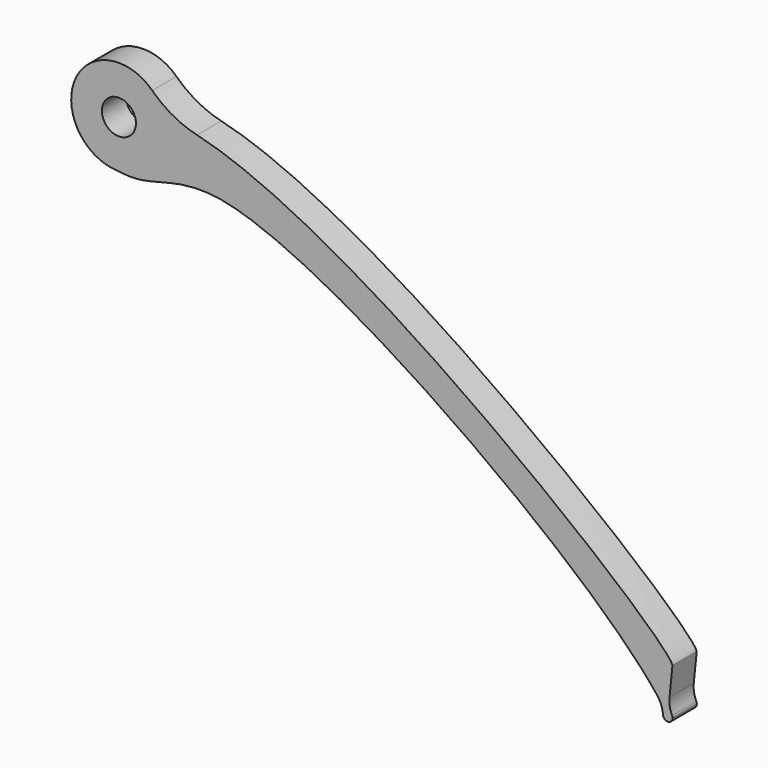
from build123d import *

# Parameters (mm, degrees)
F1_DEPTH = 3.175
F2_R     = 10
F3_R     = 5
F4_R     = 3


# Not quite as in the source:
# - a length typed as a fraction of an inch, garbled in the dataset ("3 / 203.2 mm" for 3/8 in), is restored


with BuildPart() as f1:
    # F0 (on Front) → F1 (new body)
    with BuildSketch(Plane.XZ):
        with BuildLine():
            ThreePointArc((5, 0), (4.9416586843, 0.7615835135), (4.7679962208, 1.5053943132))
            ThreePointArc((4.7679962208, 1.5053943132), (-4.0328012328, 2.9557594992), (0, -5))
            ThreePointArc((0, -5), (3.5355339059, -3.5355339059), (5, 0))
        make_face()
        with BuildLine():
            ThreePointArc((1.4790914289, 1.0009302168), (1.7075036754, 0.5234538686), (1.7859375, 0))
            ThreePointArc((1.7859375, 0), (-1.7075036754, -0.5234538686), (1.4790914289, 1.0009302168))
        make_face(mode=Mode.SUBTRACT)
        with BuildLine():
            add(Edge.make_bspline(
                [(4.7679962208, 1.5053943132), (10.5227651302, 1.3088265612), (33.1362274433, -9.6066408427), (57.5003811193, -30.0100648608), (57.9834021628, -31.7015722394)],
                knots=[0.1250018118, 0.1250018118, 0.1250018118, 0.1250018118, 0.4750790038, 1, 1, 1, 1], degree=3))
            ThreePointArc((4.7679962208, 1.5053943132), (4.9416586843, 0.7615835135), (5, 0))
            ThreePointArc((5, 0), (3.5355339059, -3.5355339059), (0, -5))
            add(Edge.make_bspline(
                [(0, -5), (3.595217635, -5.6845152728), (10.4140448254, 2.5517302892), (51.028263127, -26.9198999285), (57.2202324906, -36.1351662136)],
                knots=[0, 0, 0, 0, 0.3070952206, 0.9894399722, 0.9894399722, 0.9894399722, 0.9894399722], degree=3))
            ThreePointArc((57.2202324906, -36.1351662136), (57.3746325338, -36.0688709445), (57.5422763348, -36.0574695402))
            Line((57.5422763348, -36.0574695402), (57.9834021628, -31.7015722394))
        make_face()
        with BuildLine():
            ThreePointArc((57.5422763348, -36.0574695402), (57.3746325338, -36.0688709445), (57.2202324906, -36.1351662136))
            add(Edge.make_bspline(
                [(57.2202324906, -36.1351662136), (57.316059957, -36.2777824909), (57.40666212, -36.4177380179), (57.4918985367, -36.5549251437)],
                knots=[0.9894399722, 0.9894399722, 0.9894399722, 0.9894399722, 1, 1, 1, 1], degree=3))
            Line((57.4918985367, -36.5549251437), (57.5422763348, -36.0574695402))
        make_face()
        with BuildLine():
            add(Edge.make_bspline(
                [(57.2202324906, -36.1351662136), (57.316059957, -36.2777824909), (57.40666212, -36.4177380179), (57.4918985367, -36.5549251437)],
                knots=[0.9894399722, 0.9894399722, 0.9894399722, 0.9894399722, 1, 1, 1, 1], degree=3))
            ThreePointArc((57.2202324906, -36.1351662136), (57.2529770255, -36.9941477655), (57.9918985367, -36.5549251437))
            ThreePointArc((57.9918985367, -36.5549251437), (57.8628357949, -36.2196557737), (57.5422763348, -36.0574695402))
            Line((57.5422763348, -36.0574695402), (57.4918985367, -36.5549251437))
        make_face()
    extrude(amount=F1_DEPTH)

    # F2
    f2_edges = [f1.edges().sort_by_distance(p)[0] for p in [
        (4.767996, -1.5875, 1.505394),
    ]]
    fillet(f2_edges, radius=F2_R)

    # F3
    f3_edges = [f1.edges().sort_by_distance(p)[0] for p in [
        (0, -1.5875, -5),
    ]]
    fillet(f3_edges, radius=F3_R)

    # F4
    f4_edges = [f1.edges().sort_by_distance(p)[0] for p in [
        (57.542276, -1.5875, -36.05747),
        (57.220232, -1.5875, -36.135166),
    ]]
    fillet(f4_edges, radius=F4_R)


solid = f1.part
